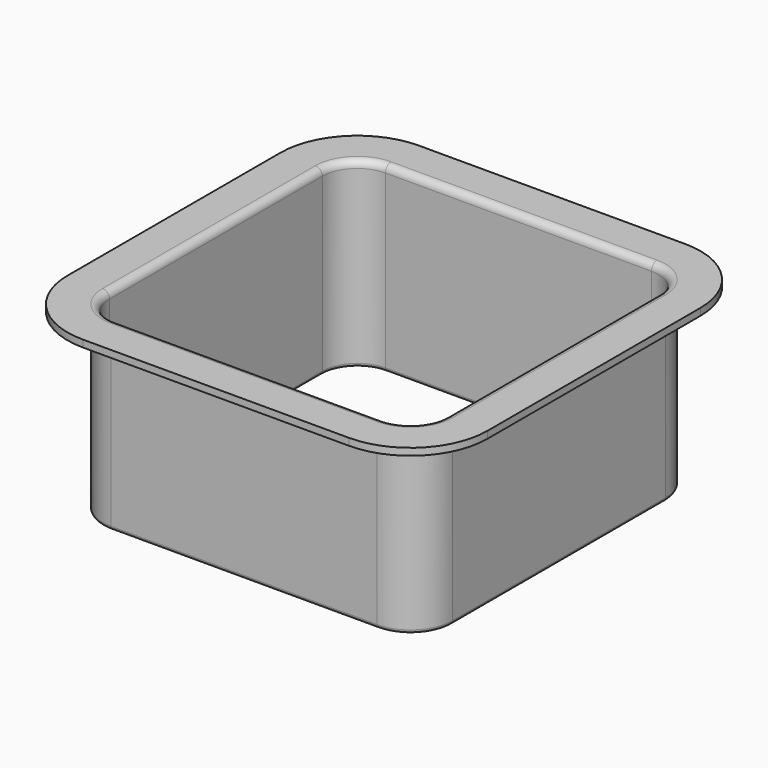
from build123d import *

# Parameters (mm, degrees)
F1_DEPTH = 2
F3_DEPTH = 50
F4_R     = 0.99999
F5_R     = 2


# Not quite as in the source:
# - a fillet or chamfer is up to 0.001 mm smaller than in the source, because OpenCascade refuses the exact size


with BuildPart() as f1:
    # F0 (on Top) → F1 (new body)
    with BuildSketch(Plane.XY):
        with BuildLine():
            Line((-67.3099028766, 44.4781833887), (-67.3099028766, -31.5218166113))
            ThreePointArc((-67.3099028766, -31.5218166113), (-60.8662520627, -47.0781657974), (-45.3099028766, -53.5218166113))
            Line((-45.3099028766, -53.5218166113), (30.6900971234, -53.5218166113))
            ThreePointArc((30.6900971234, -53.5218166113), (46.2464463095, -47.0781657974), (52.6900971234, -31.5218166113))
            Line((52.6900971234, -31.5218166113), (52.6900971234, 44.4781833887))
            ThreePointArc((52.6900971234, 44.4781833887), (46.2464463095, 60.0345325748), (30.6900971234, 66.4781833887))
            Line((30.6900971234, 66.4781833887), (-45.3099028766, 66.4781833887))
            ThreePointArc((-45.3099028766, 66.4781833887), (-60.8662520627, 60.0345325748), (-67.3099028766, 44.4781833887))
        make_face()
        with BuildLine():
            ThreePointArc((-55.3099028766, 44.4781833887), (-52.3809706885, 51.5492512006), (-45.3099028766, 54.4781833887))
            Line((-45.3099028766, 54.4781833887), (30.6900971234, 54.4781833887))
            ThreePointArc((30.6900971234, 54.4781833887), (37.7611649352, 51.5492512006), (40.6900971234, 44.4781833887))
            Line((40.6900971234, 44.4781833887), (40.6900971234, -31.5218166113))
            ThreePointArc((40.6900971234, -31.5218166113), (37.7611649352, -38.5928844232), (30.6900971234, -41.5218166113))
            Line((30.6900971234, -41.5218166113), (-45.3099028766, -41.5218166113))
            ThreePointArc((-45.3099028766, -41.5218166113), (-52.3809706885, -38.5928844232), (-55.3099028766, -31.5218166113))
            Line((-55.3099028766, -31.5218166113), (-55.3099028766, 44.4781833887))
        make_face(mode=Mode.SUBTRACT)
    extrude(amount=F1_DEPTH)

    # F2 (on Top) → F3 (join)
    with BuildSketch(Plane.XY):
        with BuildLine():
            Line((-45.3099028766, -43.5218166113), (30.6900971234, -43.5218166113))
            ThreePointArc((30.6900971234, -43.5218166113), (39.1753784976, -40.0070979855), (42.6900971234, -31.5218166113))
            Line((42.6900971234, -31.5218166113), (42.6900971234, 44.4781833887))
            ThreePointArc((42.6900971234, 44.4781833887), (39.1753784976, 52.9634647629), (30.6900971234, 56.4781833887))
            Line((30.6900971234, 56.4781833887), (-45.3099028766, 56.4781833887))
            ThreePointArc((-45.3099028766, 56.4781833887), (-53.7951842509, 52.9634647629), (-57.3099028766, 44.4781833887))
            Line((-57.3099028766, 44.4781833887), (-57.3099028766, -31.5218166113))
            ThreePointArc((-57.3099028766, -31.5218166113), (-53.7951842509, -40.0070979855), (-45.3099028766, -43.5218166113))
        make_face()
        with BuildLine():
            Line((-45.3099028766, 54.4781833887), (30.6900971234, 54.4781833887))
            ThreePointArc((30.6900971234, 54.4781833887), (37.7611649352, 51.5492512006), (40.6900971234, 44.4781833887))
            Line((40.6900971234, 44.4781833887), (40.6900971234, -31.5218166113))
            ThreePointArc((40.6900971234, -31.5218166113), (37.7611649352, -38.5928844232), (30.6900971234, -41.5218166113))
            Line((30.6900971234, -41.5218166113), (-45.3099028766, -41.5218166113))
            ThreePointArc((-45.3099028766, -41.5218166113), (-52.3809706885, -38.5928844232), (-55.3099028766, -31.5218166113))
            Line((-55.3099028766, -31.5218166113), (-55.3099028766, 44.4781833887))
            ThreePointArc((-55.3099028766, 44.4781833887), (-52.3809706885, 51.5492512006), (-45.3099028766, 54.4781833887))
        make_face(mode=Mode.SUBTRACT)
    extrude(amount=-F3_DEPTH)

    # F4 (radius 1 in the source; OpenCascade refuses exactly that, so slightly less here)
    f4_edges = [f1.edges().sort_by_distance(p)[0] for p in [
        (-55.309903, 6.478183, -50),
        (-57.309903, 6.478183, -50),
    ]]
    fillet(f4_edges, radius=F4_R)

    # F5
    f5_edges = [f1.edges().sort_by_distance(p)[0] for p in [
        (-7.309903, 54.478183, 2),
    ]]
    fillet(f5_edges, radius=F5_R)


solid = f1.part
